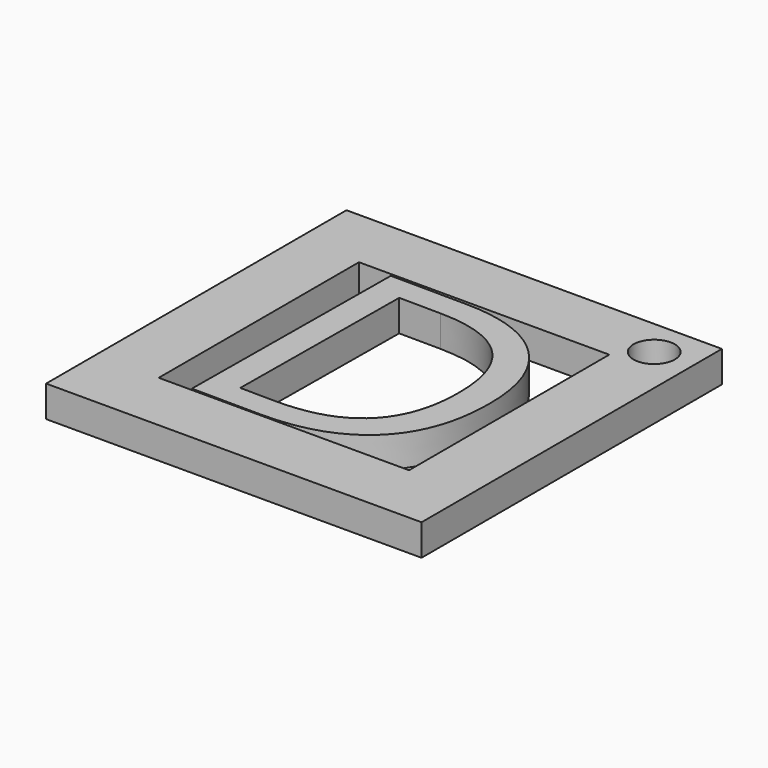
from build123d import *

# Parameters (mm, degrees)
F0_W         = 60
F0_H         = 60
F0_W_2       = 40
F0_H_2       = 40
F2_DEPTH     = 5
F1_TEXT_SIZE = 55.0634642253
F3_DEPTH     = 5
F4_R         = 3.2991727719
F5_DEPTH     = 25.4


# Not quite as in the source:
# - Text() gives the source's letters only with a copy of the font that has no kerning and outlines rounded to 1/6400 em; it was checked with that copy


with BuildPart() as f2:
    # F0 (on Top) → F2 (new body)
    with BuildSketch(Plane.XY):
        with Locations((-6.0453659881, 0.1883533943)):
            Rectangle(F0_W, F0_H)
        with Locations((-6.0453659881, 0.1883533943)):
            Rectangle(F0_W_2, F0_H_2, mode=Mode.SUBTRACT)
    extrude(amount=F2_DEPTH)

    # F4 (on face) → F5 (cut)
    with BuildSketch(Plane.XY.offset(5)):
        with Locations((17.8594775498, 24.2810193449)):
            Circle(F4_R)
    extrude(amount=-F5_DEPTH, mode=Mode.SUBTRACT)


with BuildPart() as f3:
    # F1 (on face) → F3 (new body)
    with BuildSketch(Plane.XY):
        with Locations(Location((-26.3949917691, -19.4557991854), (0, 0, -0.5052841602))):
            Text('D', F1_TEXT_SIZE, font='Open Sans', text_align=(TextAlign.LEFT, TextAlign.BOTTOM))
    extrude(amount=F3_DEPTH)


solid = Compound([f2.part, f3.part])
